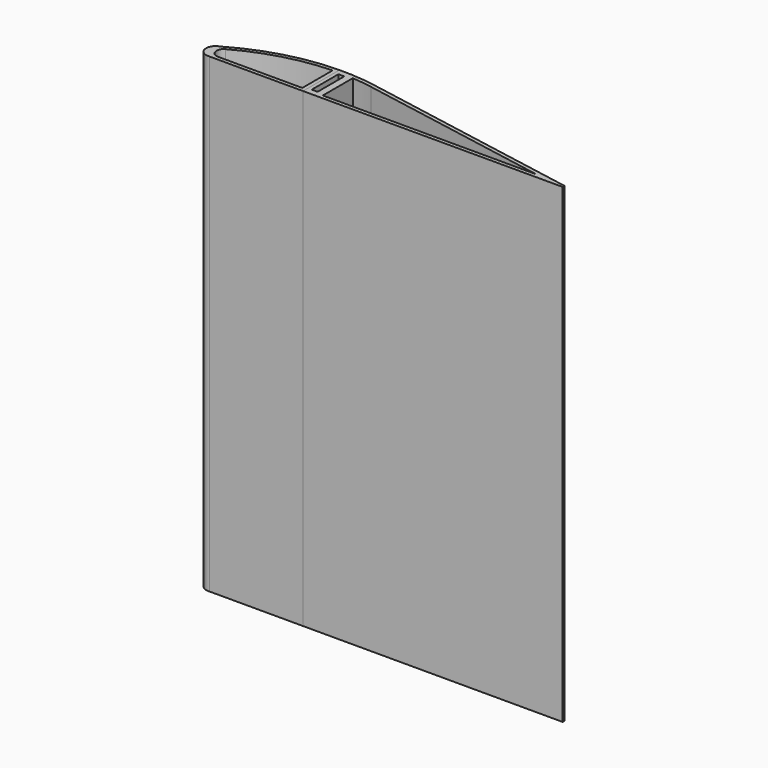
from build123d import *

# Parameters (mm, degrees)
F1_DEPTH      = 200
F3_DEPTH      = 200
F4_T          = -1.6
F4_2_T        = -1.6
F5_DEPTH      = 1.6
F6_W          = 2.5
F6_H          = 1
F7_DEPTH      = 20
F8_T4_ANGLE   = 38.4955577252
F8_T11_ANGLE  = 38.4955577252
F8_T18_ANGLE  = 38.4955577252
F8_T25_DEPTH  = 5.5
F8_T31_DEPTH  = 5.5
F8_T37_DEPTH  = 5.5
F9_W          = 1.672731913
F9_H          = 0.2267822191
F9_H_2        = 0.1519754522
F10_DEPTH     = 20
F11_T4_ANGLE  = 36.7926896337
F11_T10_ANGLE = 36.7926896337
F11_T18_DEPTH = 29.7195290041
F11_T23_DEPTH = 4.7195290041
F13_DEPTH     = 200
F14_R         = 3


# Not quite as in the source:
# - a fillet or chamfer that OpenCascade refuses, or shapes differently, is made with other operations: its cross-section is extruded or revolved along the edge and cut away or added


with BuildPart() as f1:
    # F0 (on Top) → F1 (new body)
    with BuildSketch(Plane.XY):
        with BuildLine():
            Line((94.1401966023, -3), (94.1696608117, -2.0004341641))
            Line((94.1696608117, -2.0004341641), (0, 15))
            ThreePointArc((0, 15), (-7.9879059152, 16.0504323354), (-16.0396361483, 16.3327251865))
            Line((-16.0396361483, 16.3327251865), (-16.0396361483, -3))
            Line((-16.0396361483, -3), (94.1401966023, -3))
        make_face()
    extrude(amount=F1_DEPTH)

    # F4
    f4_openings = [f1.faces().sort_by_distance(p)[0] for p in [
        (22.614044, 3.891358, 200),
    ]]
    offset(amount=F4_T, openings=f4_openings)


with BuildPart() as f3:
    # F2 (on face) → F3 (new body)
    with BuildSketch(Plane.XY.offset(200)):
        with BuildLine():
            Line((-16.0396361483, -3), (-16.0396361483, 16.3327251865))
            ThreePointArc((-16.0396361483, 16.3327251865), (-37.5222437907, 13.2612199418), (-57.5066562048, 4.8019152395))
            ThreePointArc((-57.5066562048, 4.8019152395), (-60.2806962129, 0.1415930949), (-55.8598033977, -3))
            Line((-55.8598033977, -3), (-16.0396361483, -3))
        make_face()
    extrude(amount=-F3_DEPTH)

    # F4#2
    f4_2_openings = [f3.faces().sort_by_distance(p)[0] for p in [
        (-34.83961, 5.023506, 200),
    ]]
    offset(amount=F4_2_T, openings=f4_2_openings, kind=Kind.INTERSECTION)


with BuildPart() as f5_tool:
    # F4_face (on face) → F5 (new body, through all)
    with BuildSketch(Plane(origin=(-34.5686000718, 5.0952187138, 1.6), x_dir=(1, 0, 0), z_dir=(0, 0, 1))):
        with BuildLine():
            ThreePointArc((16.9289639236, 9.600978508), (-3.4092890923, 6.3732828215), (-22.3173938219, -1.7842983593))
            ThreePointArc((-22.3173938219, -1.7842983593), (-24.1546496637, -4.5833369872), (-21.4060437384, -6.4952187138))
            Line((-21.4060437384, -6.4952187138), (16.9289639236, -6.4952187138))
            Line((16.9289639236, -6.4952187138), (16.9289639236, 9.600978508))
        make_face()
        with BuildLine():
            Line((116.4062392425, -6.4952187138), (34.2843472293, 8.3302336301))
            ThreePointArc((34.2843472293, 8.3302336301), (27.2349408421, 9.2915509636), (20.1289639236, 9.6427680764))
            Line((20.1289639236, 9.6427680764), (20.1289639236, -6.4952187138))
            Line((20.1289639236, -6.4952187138), (116.4062392425, -6.4952187138))
        make_face()
    extrude(amount=-F5_DEPTH)


with BuildPart() as f1_1:
    add(f1.part)

    # F5: cut by f5_tool
    add(f5_tool.part, mode=Mode.SUBTRACT)

    # F6 (on face) → F7 (join)
    with BuildSketch(Plane.XY.offset(200)):
        Polygon((-11.9396361483, -0.4), (-11.9396361483, -1.4), (-8.9396361483, -1.4), (-8.9396361483, 14.7379867902), (-11.9396361483, 14.7379867902), (-11.9396361483, 13.7379867902), align=None)
        with Locations((-13.1896361483, -0.9)):
            Rectangle(F6_W, F6_H)
        with Locations((-13.1896361483, 14.2379867902)):
            Rectangle(F6_W, F6_H)
    extrude(amount=-F7_DEPTH)

    # F8: fillet of radius 10 on 2 edges, made by hand


with BuildPart() as f3_1:
    add(f3.part)

    # F5: cut by f5_tool
    add(f5_tool.part, mode=Mode.SUBTRACT)

    # F12 (on face) → F13 (join)
    with BuildSketch(Plane.XY.offset(200)):
        with BuildLine():
            Line((-55.9746438103, -1.4), (-56.8859938937, 3.3109203545))
            ThreePointArc((-56.8859938937, 3.3109203545), (-58.7232497355, 0.5118817266), (-55.9746438103, -1.4))
        make_face()
    extrude(amount=-F13_DEPTH)

    # F14
    f14_edges = [f3_1.edges().sort_by_distance(p)[0] for p in [
        (-56.885994, 3.31092, 100),
        (-55.974644, -1.4, 100),
    ]]
    fillet(f14_edges, radius=F14_R)


with BuildPart() as f8_tool2:
    # F8_s3 → F8_t4 (revolve)
    with BuildSketch(Plane(origin=(10.2125694644, -4.0266529318, 0), x_dir=(0, 0, 1), z_dir=(0.9302990198, -0.3668020363, 0))):
        with BuildLine():
            ThreePointArc((170, -13.982703924), (177.0710678119, -11.0537717359), (180, -3.982703924))
            Line((180, -3.982703924), (180, -13.982703924))
            Line((180, -13.982703924), (170, -13.982703924))
        make_face()
    revolve(axis=Axis((-14.9610707823, -67.8731164952, 180), (0, 0, 1)), revolution_arc=F8_T4_ANGLE)

    split(bisect_by=Plane.YZ.offset(-8.9396361483), keep=Keep.BOTTOM)

    split(bisect_by=Plane.YZ.offset(-11.9396361483), keep=Keep.TOP)

    split(bisect_by=Plane.XZ.offset(-13.7379867902), keep=Keep.TOP)


with BuildPart() as f1_2:
    add(f1_1.part)

    # F8_t1: union F8_tool2
    add(f8_tool2.part)


with BuildPart() as f8_tool9:
    # F8_s10 → F8_t11 (revolve)
    with BuildSketch(Plane(origin=(10.2125694644, -4.0266529318, 0), x_dir=(0, 0, 1), z_dir=(0.9302990198, -0.3668020363, 0))):
        with BuildLine():
            ThreePointArc((170, -13.982703924), (177.0710678119, -11.0537717359), (180, -3.982703924))
            Line((180, -3.982703924), (180, -13.982703924))
            Line((180, -13.982703924), (170, -13.982703924))
        make_face()
    revolve(axis=Axis((-14.9610707823, -67.8731164952, 180), (0, 0, 1)), revolution_arc=F8_T11_ANGLE)

    split(bisect_by=Plane.YZ.offset(-8.9396361483), keep=Keep.BOTTOM)

    split(bisect_by=Plane.YZ.offset(-11.9396361483), keep=Keep.TOP)

    split(bisect_by=Plane.XZ.offset(-13.7379867902), keep=Keep.BOTTOM)


with BuildPart() as f1_3:
    add(f1_2.part)

    # F8_t8: union F8_tool9
    add(f8_tool9.part)


with BuildPart() as f8_tool16:
    # F8_s17 → F8_t18 (revolve)
    with BuildSketch(Plane(origin=(10.2125694644, -4.0266529318, 0), x_dir=(0, 0, 1), z_dir=(0.9302990198, -0.3668020363, 0))):
        with BuildLine():
            ThreePointArc((170, -13.982703924), (177.0710678119, -11.0537717359), (180, -3.982703924))
            Line((180, -3.982703924), (180, -13.982703924))
            Line((180, -13.982703924), (170, -13.982703924))
        make_face()
    revolve(axis=Axis((-14.9610707823, -67.8731164952, 180), (0, 0, 1)), revolution_arc=F8_T18_ANGLE)

    split(bisect_by=Plane.YZ.offset(-14.4396361483), keep=Keep.TOP)

    split(bisect_by=Plane.YZ.offset(-11.9396361483), keep=Keep.BOTTOM)

    split(bisect_by=Plane.XZ.offset(-13.7379867902), keep=Keep.BOTTOM)


with BuildPart() as f1_4:
    add(f1_3.part)

    # F8_t15: union F8_tool16
    add(f8_tool16.part)


with BuildPart() as f8_tool23:
    # F8_s24 → F8_t25 (new body)
    with BuildSketch(Plane.YZ.offset(-14.4396361483)):
        with BuildLine():
            ThreePointArc((-1.4, 170), (1.5289321881, 177.0710678119), (8.6, 180))
            Line((8.6, 180), (-1.4, 180))
            Line((-1.4, 180), (-1.4, 170))
        make_face()
    extrude(amount=F8_T25_DEPTH)

    split(bisect_by=Plane.XZ.offset(0.4), keep=Keep.TOP)

    split(bisect_by=Plane.YZ.offset(-11.9396361483), keep=Keep.BOTTOM)


with BuildPart() as f1_5:
    add(f1_4.part)

    # F8_t22: union F8_tool23
    add(f8_tool23.part)


with BuildPart() as f8_tool29:
    # F8_s30 → F8_t31 (new body)
    with BuildSketch(Plane.YZ.offset(-14.4396361483)):
        with BuildLine():
            ThreePointArc((-1.4, 170), (1.5289321881, 177.0710678119), (8.6, 180))
            Line((8.6, 180), (-1.4, 180))
            Line((-1.4, 180), (-1.4, 170))
        make_face()
    extrude(amount=F8_T31_DEPTH)

    split(bisect_by=Plane.XZ.offset(0.4), keep=Keep.TOP)

    split(bisect_by=Plane.YZ.offset(-11.9396361483), keep=Keep.TOP)


with BuildPart() as f1_6:
    add(f1_5.part)

    # F8_t28: union F8_tool29
    add(f8_tool29.part)


with BuildPart() as f8_tool35:
    # F8_s36 → F8_t37 (new body)
    with BuildSketch(Plane.YZ.offset(-14.4396361483)):
        with BuildLine():
            ThreePointArc((-1.4, 170), (1.5289321881, 177.0710678119), (8.6, 180))
            Line((8.6, 180), (-1.4, 180))
            Line((-1.4, 180), (-1.4, 170))
        make_face()
    extrude(amount=F8_T37_DEPTH)

    split(bisect_by=Plane.XZ.offset(0.4), keep=Keep.BOTTOM)

    split(bisect_by=Plane.YZ.offset(-11.9396361483), keep=Keep.TOP)


with BuildPart() as f1_7:
    add(f1_6.part)

    # F8_t34: union F8_tool35
    add(f8_tool35.part)

    # F9 (on face) → F10 (join)
    with BuildSketch(Plane(origin=(0, 0, 0), x_dir=(1, 0, 0), z_dir=(0, 0, -1))):
        Polygon((-9.7201071442, -14.7104891011), (-9.7201071442, 1.4), (-12.7669042352, 1.4), (-12.7669042352, 1.1732177809), (-12.7669042352, -14.5585136488), (-12.7669042352, -14.7104891011), align=None)
        with Locations((-13.6032701918, 1.2866088904)):
            Rectangle(F9_W, F9_H)
        with Locations((-13.6032701918, -14.6345013749)):
            Rectangle(F9_W, F9_H_2)
    extrude(amount=-F10_DEPTH)

    # F11: fillet of radius 10 on 2 edges, made by hand


with BuildPart() as f11_tool2:
    # F11_s3 → F11_t4 (revolve)
    with BuildSketch(Plane(origin=(9.6429632601, -3.6969453305, 0), x_dir=(0, 0, 1), z_dir=(0.9337307092, -0.3579762042, 0))):
        with BuildLine():
            ThreePointArc((30, -13.8818283686), (22.9289321881, -10.9528961805), (20, -3.8818283686))
            Line((20, -3.8818283686), (20, -13.8818283686))
            Line((20, -13.8818283686), (30, -13.8818283686))
        make_face()
    revolve(axis=Axis((-14.9610707823, -67.8731164952, 20), (0, 0, 1)), revolution_arc=F11_T4_ANGLE)

    split(bisect_by=Plane.YZ.offset(-12.7669042352), keep=Keep.TOP)

    split(bisect_by=Plane.YZ.offset(-9.7201071442), keep=Keep.BOTTOM)


with BuildPart() as f1_8:
    add(f1_7.part)

    # F11_t1: union F11_tool2
    add(f11_tool2.part)


with BuildPart() as f11_tool8:
    # F11_s9 → F11_t10 (revolve)
    with BuildSketch(Plane(origin=(9.6429632601, -3.6969453305, 0), x_dir=(0, 0, 1), z_dir=(0.9337307092, -0.3579762042, 0))):
        with BuildLine():
            ThreePointArc((30, -13.8818283686), (22.9289321881, -10.9528961805), (20, -3.8818283686))
            Line((20, -3.8818283686), (20, -13.8818283686))
            Line((20, -13.8818283686), (30, -13.8818283686))
        make_face()
    revolve(axis=Axis((-14.9610707823, -67.8731164952, 20), (0, 0, 1)), revolution_arc=F11_T10_ANGLE)

    split(bisect_by=Plane.YZ.offset(-14.4396361483), keep=Keep.TOP)

    split(bisect_by=Plane.XZ.offset(-14.5585136488), keep=Keep.BOTTOM)

    split(bisect_by=Plane.XZ.offset(-14.7104891011), keep=Keep.TOP)

    split(bisect_by=Plane.YZ.offset(-9.7201071442), keep=Keep.BOTTOM)


with BuildPart() as f1_9:
    add(f1_8.part)

    # F11_t7: union F11_tool8
    add(f11_tool8.part)


with BuildPart() as f11_tool16:
    # F11_s17 → F11_t18 (new body)
    with BuildSketch(Plane.YZ.offset(-9.7201071442)):
        with BuildLine():
            ThreePointArc((-1.4, 30), (1.5289321881, 22.9289321881), (8.6, 20))
            Line((8.6, 20), (-1.4, 20))
            Line((-1.4, 20), (-1.4, 30))
        make_face()
    extrude(amount=-F11_T18_DEPTH)

    split(bisect_by=Plane.YZ.offset(-12.7669042352), keep=Keep.TOP)


with BuildPart() as f1_10:
    add(f1_9.part)

    # F11_t15: union F11_tool16
    add(f11_tool16.part)


with BuildPart() as f11_tool21:
    # F11_s22 → F11_t23 (new body)
    with BuildSketch(Plane.YZ.offset(-9.7201071442)):
        with BuildLine():
            ThreePointArc((-1.4, 30), (1.5289321881, 22.9289321881), (8.6, 20))
            Line((8.6, 20), (-1.4, 20))
            Line((-1.4, 20), (-1.4, 30))
        make_face()
    extrude(amount=-F11_T23_DEPTH)

    split(bisect_by=Plane.XZ.offset(1.1732177809), keep=Keep.TOP)


with BuildPart() as f1_11:
    add(f1_10.part)

    # F11_t20: union F11_tool21
    add(f11_tool21.part)


solid = Compound([f3_1.part, f1_11.part])
